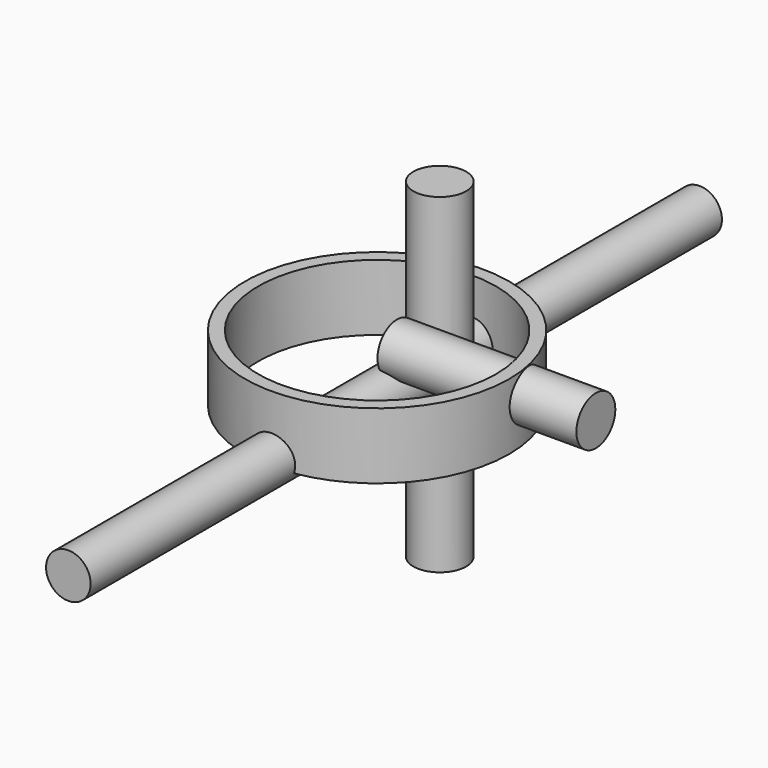
from build123d import *

# Parameters (mm, degrees)
F0_R     = 50.8
F1_DEPTH = 25.4
F2_T     = -5.08
F3_R     = 8.5698519832
F4_DEPTH = 148.336
F5_DEPTH = 154.94
F6_R     = 10.165051904
F7_DEPTH = 63.5
F8_R     = 9.3473873545
F9_DEPTH = 76.454


with BuildPart() as f1:
    # F0 (on Top) → F1 (new body)
    with BuildSketch(Plane.XY):
        Circle(F0_R)
    extrude(amount=F1_DEPTH)

    # F2
    f2_openings = [f1.faces().sort_by_distance(p)[0] for p in [
        (0, 0, 25.4),
        (0, 0, 0),
    ]]
    offset(amount=F2_T, openings=f2_openings)


with BuildPart() as f4:
    # F3 (on Front) → F4 (new body)
    with BuildSketch(Plane.XZ):
        with Locations((0, 2.6629630011)):
            Circle(F3_R)
    extrude(amount=F4_DEPTH)

    # F3 (on Front) → F5 (join)
    with BuildSketch(Plane.XZ):
        with Locations((0, 2.6629630011)):
            Circle(F3_R)
    extrude(amount=-F5_DEPTH)

    # F6 (on Top) → F7 (join, symmetric)
    with BuildSketch(Plane.XY):
        with Locations((0, 30.111702159)):
            Circle(F6_R)
    extrude(amount=F7_DEPTH, both=True)


with BuildPart() as f9:
    # F8 (on Right) → F9 (new body)
    with BuildSketch(Plane.YZ):
        with Locations((9.5232129097, 15.795622021)):
            Circle(F8_R)
    extrude(amount=F9_DEPTH)


with BuildPart() as f1_1:
    add(f1.part)

    # F10: cut F4
    add(f4.part, mode=Mode.SUBTRACT)

    # F11: cut F9
    add(f9.part, mode=Mode.SUBTRACT)


solid = Compound([f4.part, f9.part, f1_1.part])
